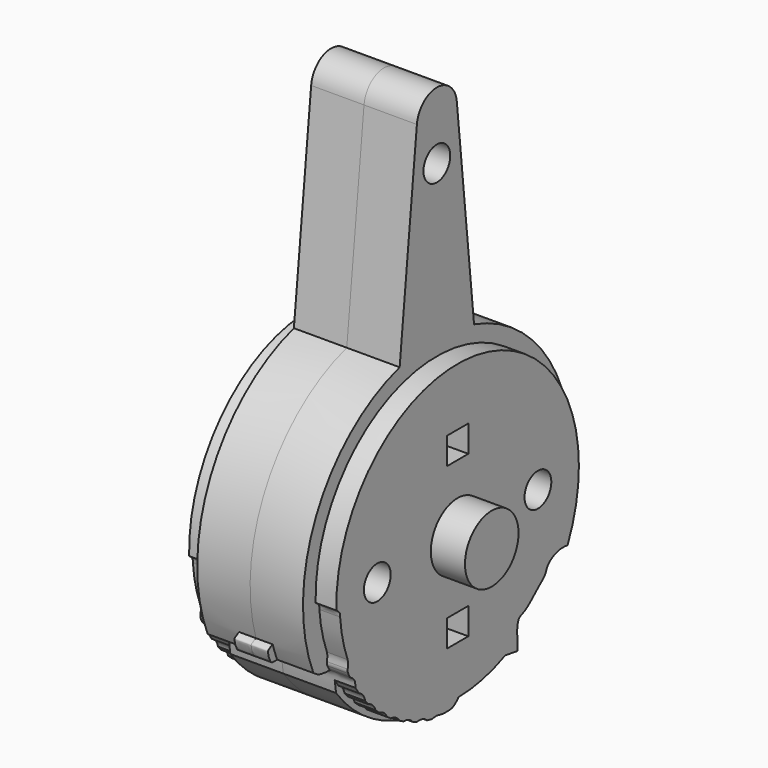
from build123d import *

# Parameters (mm, degrees)
F1_DEPTH          = 10.033
F2_R              = 28.7655
F3_DEPTH          = 13.97
F4_R              = 6.35
F5_DEPTH          = 20.447
F7_DEPTH          = 13.971
F9_DEPTH          = 3.175
F12_DEPTH         = 19.178
F13_R             = 0.9578377191
F14_DEPTH         = 1.2710025
F15_R             = 1.27
F18_DEPTH         = 3.937
F19_R             = 1.27
F20_R             = 2.54
F21_DEPTH         = 3.937
F21_COPIES_COUNT  = 6
F21_COPIES_ANGLE  = 35
F23_W             = 5.08
F23_H             = 5.08
F24_DEPTH         = 20.448
F24_DEPTH_BACK    = 20.448
F26_D             = 3.683
F26_CBORE_D       = 6.35
F26_CBORE_DEPTH   = 6.35
F26_2_D           = 3.683
F26_2_CBORE_D     = 6.35
F26_2_CBORE_DEPTH = 6.35
F28_D             = 3.683
F28_CBORE_D       = 6.35
F28_CBORE_DEPTH   = 6.35
F28_2_D           = 3.683
F28_2_CBORE_D     = 6.35
F28_2_CBORE_DEPTH = 6.35
F29_R             = 1.8415
F30_DEPTH         = 6.35


# Not quite as in the source:
# - a pattern or mirror of a feature is missing from the dataset's text; its kind, count and spacing are read off the source's solid


with BuildPart() as f1:
    # F0 (on Right) → F1 (new body)
    with BuildSketch(Plane.YZ):
        with BuildLine():
            Line((-4.7364105267, 69.3953168063), (-8.8245775918, 30.499005399))
            ThreePointArc((-8.8245775918, 30.499005399), (-28.5184027319, -13.9557588694), (18.6681298638, -25.6819669688))
            Line((18.6681298638, -25.6819669688), (25.6109423935, -26.769625023))
            Line((25.6109423935, -26.769625023), (27.2527408148, -16.2895861851))
            ThreePointArc((27.2527408148, -16.2895861851), (29.5412643849, 11.6351277836), (8.8245775918, 30.499005399))
            Line((8.8245775918, 30.499005399), (4.7364105267, 69.3953168063))
            ThreePointArc((4.7364105267, 69.3953168063), (0, 73.66), (-4.7364105267, 69.3953168063))
        make_face()
    extrude(amount=F1_DEPTH)

    # F2 (on Right) → F3 (join)
    with BuildSketch(Plane.YZ):
        Circle(F2_R)
    extrude(amount=F3_DEPTH)

    # F4 (on Right) → F5 (join)
    with BuildSketch(Plane.YZ):
        Circle(F4_R)
    extrude(amount=F5_DEPTH)

    # F6 (on face) → F7 (cut, through all)
    with BuildSketch(Plane.YZ.offset(13.97)):
        with BuildLine():
            add(Edge.make_bspline(
                [(-7.1486304514, -28.9243403822), (-6.8878250908, -28.7659776031), (-6.4529218553, -28.5018648874), (-6.2231233428, -28.2128033358), (-5.8855347549, -28.061145391), (-5.5430396368, -28.030903798), (-4.9850544415, -27.9574044918), (-4.2988182622, -28.1357210395), (-3.3427062978, -28.3348289714), (-2.2855183683, -28.2786024882), (-1.3464257856, -28.2881054853), (-0.5340970307, -27.7787568653), (0.0411322385, -27.2351744219), (0.1811513888, -26.9986631251)],
                knots=[0, 0, 0, 0, 0.0984856257, 0.1633300981, 0.2265308166, 0.290124721, 0.3698982453, 0.4611289236, 0.5684094096, 0.680563766, 0.7838042297, 0.8899315192, 1, 1, 1, 1], degree=3))
            ThreePointArc((-7.1486304514, -28.9243403822), (-16.4914069902, -24.8143885551), (-23.8988204948, -17.7923231433))
            add(Edge.make_bspline(
                [(-29.288378286, -12.2577892533), (-29.093742234, -12.3776731722), (-28.7038530201, -12.6177524101), (-28.1423483443, -13.0048277861), (-27.4288144297, -13.1952282475), (-26.8979324438, -13.2355025143), (-26.0550589917, -13.4001143408), (-25.8381698833, -13.3157478239), (-25.4563424256, -13.3593485335), (-25.0612221982, -13.4767549513), (-24.7541348918, -13.8348185133), (-24.4297686006, -14.1769650028), (-24.3281607063, -14.5068300952), (-24.2682325051, -14.8181950587), (-24.2741751453, -15.1051985457), (-24.2142388772, -15.5390388554), (-24.1440327898, -16.239357365), (-24.0315701813, -16.9547982514), (-23.8988204948, -17.7923231433)],
                knots=[0, 0, 0, 0, 0.0710167377, 0.1422255366, 0.2141922301, 0.2798246298, 0.3573206116, 0.3985310067, 0.4499171356, 0.5048208114, 0.563458388, 0.6222418907, 0.6721949363, 0.7198246934, 0.7654446161, 0.8212962205, 0.8888854676, 1, 1, 1, 1], degree=3))
            ThreePointArc((-29.288378286, -12.2577892533), (-8.5585954438, -30.5747108576), (18.6681298638, -25.6819669688))
            Line((18.6681298638, -25.6819669688), (11.2888878459, -24.5259380569))
            ThreePointArc((11.2888878459, -24.5259380569), (5.8667744398, -26.3541568645), (0.1811513888, -26.9986631251))
        make_face()
    extrude(amount=-F7_DEPTH, mode=Mode.SUBTRACT)

    # F8 (on Right) → F9 (join)
    with BuildSketch(Plane.YZ):
        with BuildLine():
            add(Edge.make_bspline(
                [(-29.9831703305, -9.3742739409), (-30.3077596207, -9.1092490231), (-30.950178697, -9.5600446496), (-31.5814584915, -9.845088059), (-31.397559135, -10.4131121926), (-31.3506657225, -11.0081444142), (-31.0184240833, -11.5062042348), (-30.8571996048, -12.1462653467), (-30.1302969147, -12.299307641), (-29.3746552787, -12.2158103383), (-28.8324718743, -12.3970693619), (-29.4244788433, -9.8304416889), (-29.9831703305, -9.3742739409)],
                knots=[0, 0, 0, 0, 0.114226262, 0.2046892752, 0.2845093856, 0.3735086544, 0.4618835558, 0.549804437, 0.6439818773, 0.745990287, 0.8033908014, 1, 1, 1, 1], degree=3))
        make_face()
    extrude(amount=F9_DEPTH)

    # F11 (on offset) → F12 (cut, through all)
    with BuildSketch(Plane.YZ.offset(1.27)):
        with BuildLine():
            Line((14.247251503, -24.9893940475), (25.6109423935, -26.769625023))
            Line((25.6109423935, -26.769625023), (27.2527408148, -16.2895861851))
            ThreePointArc((27.2527408148, -16.2895861851), (27.8894068179, -15.1737763047), (28.4804129658, -14.0331242885))
            Line((28.4804129658, -14.0331242885), (26.0774529986, -12.141681735))
            add(Edge.make_bspline(
                [(26.0774529986, -12.141681735), (25.4376484697, -12.0627275228), (24.0452989027, -11.8909065082), (21.2296842728, -13.2260586426), (20.9431223528, -14.9881378702), (19.2002905979, -16.1982028671), (17.3054504487, -18.0765602272), (15.6817158692, -19.1992112069), (13.8821146816, -19.5950246386), (14.1017888209, -22.840392916), (14.247251503, -24.9893940475)],
                knots=[0, 0, 0, 0, 0.1165631814, 0.2536660617, 0.3565324896, 0.4720802912, 0.6070112732, 0.7208303047, 0.8151408593, 1, 1, 1, 1], degree=3))
        make_face()
    extrude(amount=F12_DEPTH, mode=Mode.SUBTRACT)

    # F13 (on face) → F14 (cut, through all)
    with BuildSketch(Plane.YZ.offset(1.27)):
        with Locations((23.7776264548, -20.1487075537)):
            Circle(F13_R)
    extrude(amount=-F14_DEPTH, mode=Mode.SUBTRACT)

    # F15
    f15_edges = [f1.edges().sort_by_distance(p)[0] for p in [
        (0.635, 25.610942, -26.769625),
    ]]
    fillet(f15_edges, radius=F15_R)

    # F17 (on face) → F18 (cut, through all)
    with BuildSketch(Plane.YZ.offset(13.97)):
        with BuildLine():
            add(Edge.make_bspline(
                [(-28.7558352468, -0.7456068052), (-28.4414426177, -0.9687028896), (-27.8590592903, -1.3819677944), (-27.8624849414, -1.9536589854), (-27.864061296, -2.2167295683)],
                knots=[0, 0, 0, 0, 0.539837963, 1, 1, 1, 1], degree=3))
            ThreePointArc((-28.7558352468, -0.7456068052), (-28.0162945829, -6.5223636891), (-26.1283490265, -12.0317649329))
            add(Edge.make_bspline(
                [(-26.0811871115, -10.0544259279), (-26.0526724089, -10.1619919608), (-25.9878123989, -10.4066634227), (-25.9556396916, -10.9891954899), (-26.0648832689, -11.6486503804), (-26.1283490265, -12.0317649329)],
                knots=[0, 0, 0, 0, 0.2474189542, 0.5627832098, 1, 1, 1, 1], degree=3))
            ThreePointArc((-26.0811871115, -10.0544259279), (-27.2558219009, -6.1999979349), (-27.864061296, -2.2167295683))
        make_face()
    extrude(amount=-F18_DEPTH, mode=Mode.SUBTRACT)

    # F19
    f19_edges = [f1.edges().sort_by_distance(p)[0] for p in [
        (12.0015, -26.128349, -12.031765),
        (12.0015, -25.470241, -13.36865),
    ]]
    fillet(f19_edges, radius=F19_R)

    # F20 (on face) → F21 (cut, through all)
    with BuildSketch(Plane.YZ.offset(13.97)):
        with Locations((-9.0600143859, -29.6339717778)):
            Circle(F20_R)
    f21 = extrude(amount=-F21_DEPTH, mode=Mode.SUBTRACT)

    # F21_copies: F21 ×6 about axis
    f21_copies_axis = Axis((0, 0, 0), (-1, 0, 0))
    for i in range(1, F21_COPIES_COUNT):
        add(f21.rotate(f21_copies_axis, i * F21_COPIES_ANGLE / (F21_COPIES_COUNT - 1)), mode=Mode.SUBTRACT)


with BuildPart() as f22_1:
    # F22: instance of F1
    add(f1.part.mirror(Plane.YZ))


with BuildPart() as f24_tool:
    # F23 (on Right) → F24 (new body, two sides)
    with BuildSketch(Plane.YZ) as f24_sk:
        with Locations((0, 15.24)):
            Rectangle(F23_W, F23_H)
        with Locations((0, -15.24)):
            Rectangle(F23_W, F23_H)
    extrude(amount=-F24_DEPTH)
    extrude(f24_sk.sketch, amount=F24_DEPTH_BACK)


with BuildPart() as f1_1:
    add(f1.part)

    # F24: cut by f24_tool
    add(f24_tool.part, mode=Mode.SUBTRACT)

    # F26 (through all)
    with Locations(Plane.YZ.offset(13.97)):
        with Locations((-19.05, 0)):
            f26 = CounterBoreHole(F26_D / 2, F26_CBORE_D / 2, F26_CBORE_DEPTH)

    # F26_copies: F26 across plane
    add(f26.mirror(Plane.ZX), mode=Mode.SUBTRACT)

    # F28 (through all)
    with Locations(Plane.YZ.offset(10.033)):
        with Locations((0, 60.96)):
            CounterBoreHole(F28_D / 2, F28_CBORE_D / 2, F28_CBORE_DEPTH)


with BuildPart() as f22_1_1:
    add(f22_1.part)

    # F24: cut by f24_tool
    add(f24_tool.part, mode=Mode.SUBTRACT)

    # F26#2 (through all)
    with Locations(Plane.YZ.offset(13.97)):
        with Locations((-19.05, 0)):
            f26_2 = CounterBoreHole(F26_2_D / 2, F26_2_CBORE_D / 2, F26_2_CBORE_DEPTH)

    # F26_2_copies: F26#2 across plane
    add(f26_2.mirror(Plane.ZX), mode=Mode.SUBTRACT)

    # F28#2 (through all)
    with Locations(Plane.YZ.offset(10.033)):
        with Locations((0, 60.96)):
            CounterBoreHole(F28_2_D / 2, F28_2_CBORE_D / 2, F28_2_CBORE_DEPTH)

    # F29 (on face) → F30 (cut)
    with BuildSketch(Plane(origin=(-10.033, 0, 0), x_dir=(0, -1, 0), z_dir=(-1, 0, 0))):
        Polygon((0, 56.6504030359), (3.732220451, 58.8052015179), (3.732220451, 63.1147984821), (0, 65.2695969641), (-3.732220451, 63.1147984821), (-3.732220451, 58.8052015179), align=None)
        with Locations((0, 60.96)):
            Circle(F29_R, mode=Mode.SUBTRACT)
    extrude(amount=-F30_DEPTH, mode=Mode.SUBTRACT)


solid = Compound([f1_1.part, f22_1_1.part])
